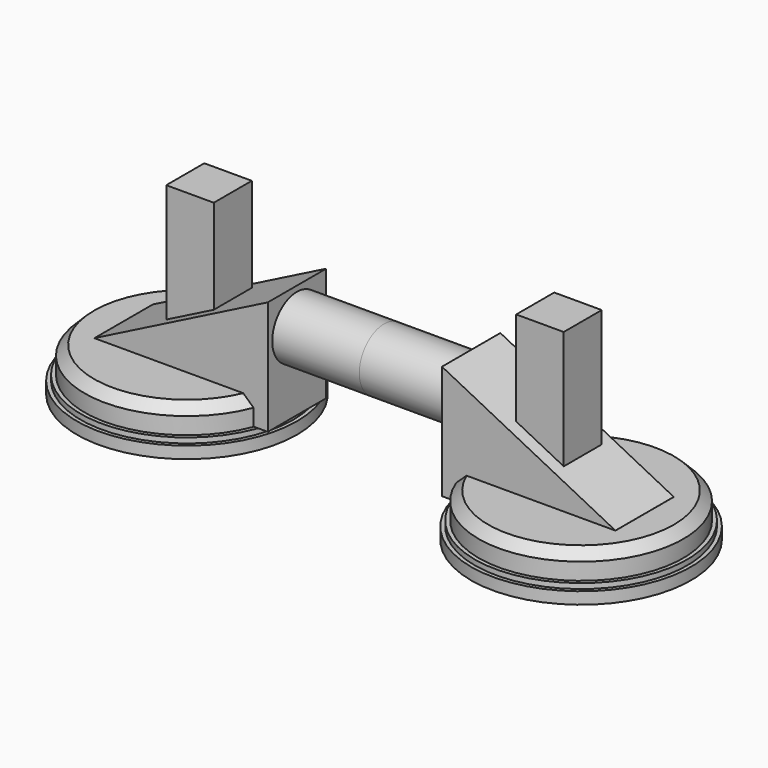
from build123d import *

# Parameters (mm, degrees)
F0_R      = 58.801
F1_DEPTH  = 6.35
F3_R      = 56.769
F4_DEPTH  = 2.794
F5_R      = 54.6989
F6_DEPTH  = 14.0716
F7_SIZE   = 5.08
F9_DEPTH  = 38.989
F10_R     = 16.51
F11_DEPTH = 46.5455
F12_W     = 25.4
F12_H     = 80.01
F13_DEPTH = 12.7


# Not quite as in the source:
# - a length typed as a fraction of an inch, garbled in the dataset ("3 / 203.2 mm" for 3/8 in), is restored


with BuildPart() as f1:
    # F0 (on Top) → F1 (new body)
    with BuildSketch(Plane.XY):
        with Locations((-105.3465, 0)):
            Circle(F0_R)
    extrude(amount=F1_DEPTH)

    # F3 (on face) → F4 (join)
    with BuildSketch(Plane.XY.offset(6.35)):
        with Locations((-105.3465, 0)):
            Circle(F3_R)
    extrude(amount=F4_DEPTH)

    # F5 (on face) → F6 (join)
    with BuildSketch(Plane.XY.offset(9.144)):
        with Locations((-105.3465, 0)):
            Circle(F5_R)
    extrude(amount=F6_DEPTH)

    # F7
    f7_edges = [f1.edges().sort_by_distance(p)[0] for p in [
        (-160.0454, 0, 23.2156),
    ]]
    chamfer(f7_edges, length=F7_SIZE)

    # F8 (on offset) → F9 (join)
    with BuildSketch(Plane.XZ.offset(19.431)):
        Polygon((-139.2555, 9.271), (-46.5455, 9.271), (-46.5455, 70.231), (-139.2555, 23.241), align=None)
    extrude(amount=-F9_DEPTH)

    # F10 (on Right) → F11 (join, through all)
    with BuildSketch(Plane.YZ):
        with Locations((0, 50.8)):
            Circle(F10_R)
    extrude(amount=-F11_DEPTH)

    # F12 (on Front) → F13 (join, symmetric)
    with BuildSketch(Plane.XZ):
        with Locations((-93.5355, 63.2206)):
            Rectangle(F12_W, F12_H)
    extrude(amount=F13_DEPTH, both=True)

    # F14: F1 across plane


with BuildPart() as f1_1:
    add(f1.part)
    add(f1.part.mirror(Plane.YZ))


solid = f1_1.part
